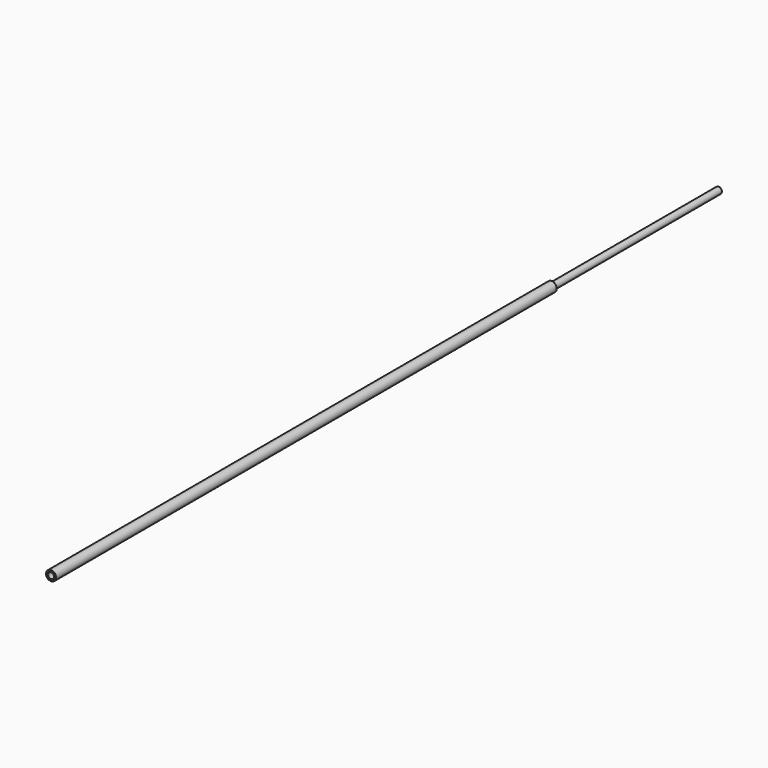
from build123d import *

# Parameters (mm, degrees)
F6_R     = 0.795
F6_R_2   = 0.7
F7_DEPTH = 150
F6_R_3   = 1.2
F6_R_4   = 0.9


# Not quite as in the source:
# - a feature of the source that left no trace in its solid (it failed there, or was rolled back) is left out
# - a pattern or mirror of a feature is missing from the dataset's text; its kind, count and spacing are read off the source's solid
# - a feature names something its author has since deleted; it is built from what else it names


with BuildPart() as f7:
    # F6 (on face) → F7 (new body)
    with BuildSketch(Plane(origin=(0, -50, 0), x_dir=(-1, 0, 0), z_dir=(0, 1, 0))):
        Circle(F6_R)
        Circle(F6_R_2, mode=Mode.SUBTRACT)
    extrude(amount=-F7_DEPTH)

    # F7_copies: F7 across plane


with BuildPart() as f7b:
    # F6 (on face) → F7, piece 2 (new body)
    with BuildSketch(Plane(origin=(0, -50, 0), x_dir=(-1, 0, 0), z_dir=(0, 1, 0))):
        Circle(F6_R_3)
        Circle(F6_R_4, mode=Mode.SUBTRACT)
    extrude(amount=-F7_DEPTH)


with BuildPart() as f7_1:
    add(f7.part)
    add(f7.part.mirror(Plane.ZX.offset(-100)))


with BuildPart() as f7b_1:
    # F10: moved
    add(f7b.part)


solid = Compound([f7_1.part, f7b_1.part])
